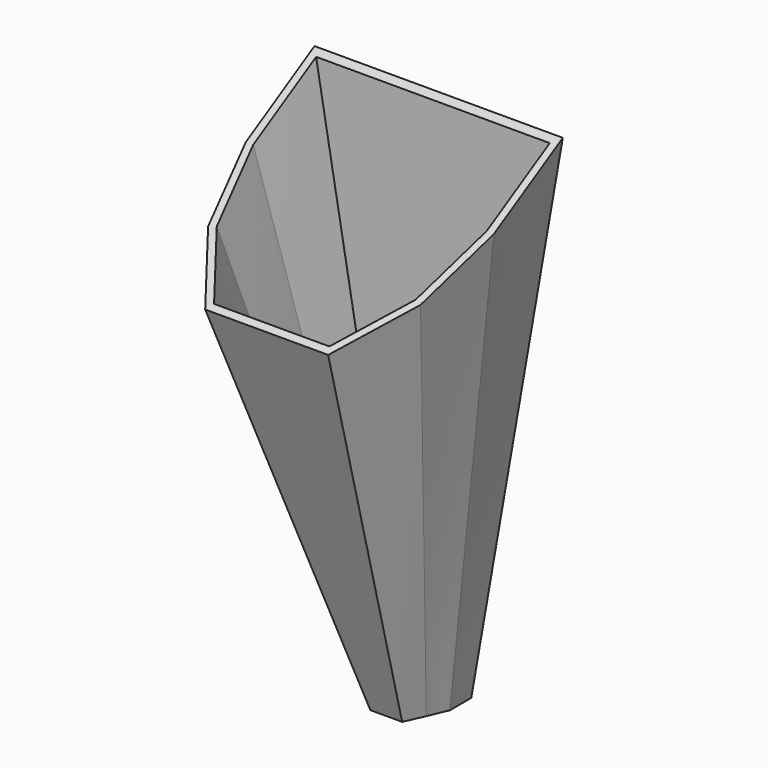
from build123d import *

# Parameters (mm, degrees)
F6_T      = 2
F8_DEPTH  = 2
F10_DEPTH = 2


# Not quite as in the source:
# - a shell that OpenCascade refuses in one call is made with other operations: the cavity is built on its own and cut out


with BuildPart() as f5:
    # F2 (on line) → F5 section 0
    with BuildSketch(Plane(origin=(0, 0, 0), x_dir=(1, 0, 0), z_dir=(0, 0.5, -0.866025))):
        Polygon((-35, 28), (-35, 0), (35, 0), (35, 28), (29.981577, 50.599864), (17.349352, 70), (0, 70), (-17.349352, 70), (-29.981577, 50.599864), align=None)
    # F4 (on offset) → F5 section 1
    with BuildSketch(Plane.XY.offset(-150)):
        Polygon((0, 0), (-8.75, 0), (-8.75, -7.25), (-6.479393, -12.375), (-4.208787, -17.5), (0, -17.5), (4.208787, -17.5), (6.479393, -12.375), (8.75, -7.25), (8.75, 0), align=None)
    loft()

    # F6: shell of thickness 2, made by hand


with BuildPart() as f6_core1:
    # F6_t2: copy of F5
    add(f5.part)

    # the walls: a layer under each face that stays
    f6_faces = [f6_core1.faces().sort_by_distance(p)[0] for p in [
        (-20.052743, -21.92362, -84.824983),
        (-14.504777, -33.579386, -90.074983),
        (-5.389535, -39.060889, -92.5),
        (5.389535, -39.060889, -92.5),
        (14.504777, -33.579386, -90.074983),
        (20.052743, -21.92362, -84.824983),
        (21.875, -7.874678, -78.5),
        (6.566526, 0, -73.234368),
        (1.479563, -7.196358, -150),
        (-21.875, -7.874678, -78.5),
        (2.162772, -22.900992, -13.221894),
    ]]
    thicken(f6_faces, amount=-F6_T, mode=Mode.SUBTRACT)


with BuildPart() as f5_1:
    add(f5.part)

    # what is left inside the walls is the cavity
    f6_cavity = [f6_core1.part.solids().sort_by_distance(p)[0] for p in [
        (4.131182, -2.02, -49.537849),
    ]]
    add(f6_cavity, mode=Mode.SUBTRACT)

    # F7 (on face) → F8 (cut)
    with BuildSketch(Plane(origin=(0, 0, 0), x_dir=(1, 0, 0), z_dir=(0, -0.5, 0.866025))):
        Polygon((45, -29.096918), (45, 10), (-45, 10), (-45, -29.096918), (-39.35082, -54.537321), (-22.771024, -80), (22.771024, -80), (39.35082, -54.537321), align=None)
        Polygon((29.981577, -50.599864), (17.349352, -70), (0, -70), (-17.349352, -70), (-29.981577, -50.599864), (-35, -28), (-35, 0), (35, 0), (35, -28), align=None, mode=Mode.SUBTRACT)
        Polygon((0, -70), (17.349352, -70), (29.981577, -50.599864), (35, -28), (35, 0), (-35, 0), (-35, -28), (-29.981577, -50.599864), (-17.349352, -70), align=None)
    extrude(amount=-F8_DEPTH, mode=Mode.SUBTRACT)

    # F9 (on face) → F10 (cut)
    with BuildSketch(Plane(origin=(0, 0, -150), x_dir=(1, 0, 0), z_dir=(0, 0, -1))):
        Polygon((15.62225, 16.425699), (15.19832, 17.382555), (10.715834, 27.5), (-10.715834, 27.5), (-15.62225, 16.425699), (-18.75, 9.366037), (-18.75, -10), (18.75, -10), (18.75, 9.366037), (15.669426, 16.319218), align=None)
        Polygon((-8.75, 0), (-8.75, 7.25), (-6.479393, 12.375), (-4.208787, 17.5), (0, 17.5), (4.208787, 17.5), (6.479393, 12.375), (6.699232, 11.878801), (8.75, 7.25), (8.75, 0), align=None, mode=Mode.SUBTRACT)
        Polygon((-6.479393, 12.375), (-8.75, 7.25), (-8.75, 0), (8.75, 0), (8.75, 7.25), (6.699232, 11.878801), (6.479393, 12.375), (4.208787, 17.5), (0, 17.5), (-4.208787, 17.5), align=None)
    extrude(amount=-F10_DEPTH, mode=Mode.SUBTRACT)


solid = f5_1.part
